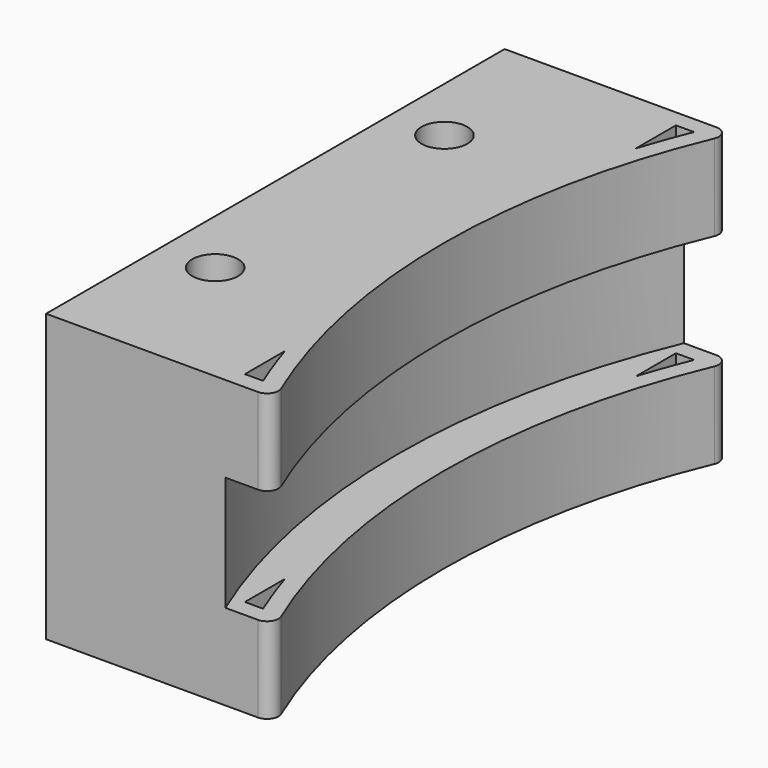
from build123d import *

# Parameters (mm, degrees)
F0_W     = 14.641710973
F0_H     = 25
F0_R     = 2
F2_DEPTH = 25
F1_W     = 8
F1_H     = 10
F4_R     = 1


# Not quite as in the source:
# - a feature names something its author has since deleted; it is built from what else it names


with BuildPart() as f2:
    # F0 (on Top) → F2 (new body)
    with BuildSketch(Plane.XY):
        with BuildLine():
            ThreePointArc((-61, 0), (-59.6453869522, 12.7838888967), (-55.641710973, 25))
            Line((-55.641710973, 25), (-61, 25))
            Line((-61, 25), (-61, 0))
        make_face()
        with BuildLine():
            Line((-59.5, 19.1311264697), (-59.5, 23.5))
            Line((-59.5, 23.5), (-57.9137289423, 23.5))
            ThreePointArc((-57.9137289423, 23.5), (-58.7474910104, 21.3303141089), (-59.5, 19.1311264697))
        make_face(mode=Mode.SUBTRACT)
        with BuildLine():
            ThreePointArc((-55.641710973, -25), (-59.6453869522, -12.7838888967), (-61, 0))
            Line((-61, 0), (-61, -25))
            Line((-61, -25), (-55.641710973, -25))
        make_face()
        with BuildLine():
            Line((-57.9137289423, -23.5), (-59.5, -23.5))
            Line((-59.5, -23.5), (-59.5, -19.1311264697))
            ThreePointArc((-59.5, -19.1311264697), (-58.7474910104, -21.3303141089), (-57.9137289423, -23.5))
        make_face(mode=Mode.SUBTRACT)
        with Locations((-68.3208554865, -12.5)):
            Rectangle(F0_W, F0_H)
        with Locations((-70.891710973, -12.5)):
            Circle(F0_R, mode=Mode.SUBTRACT)
        with Locations((-68.3208554865, 12.5)):
            Rectangle(F0_W, F0_H)
        with Locations((-70.891710973, 12.5)):
            Circle(F0_R, mode=Mode.SUBTRACT)
    extrude(amount=F2_DEPTH)

    # F1 (on Front) → F3 (revolve, cut)
    with BuildSketch(Plane.XZ):
        with Locations((-61, 12.5)):
            Rectangle(F1_W, F1_H)
    revolve(axis=Axis((0, 0, 15.2043728158), (0, 0, 1)), mode=Mode.SUBTRACT)

    # F4
    f4_edges = [f2.edges().sort_by_distance(p)[0] for p in [
        (-55.641711, 25, 21.25),
        (-55.641711, 25, 3.75),
        (-55.641711, -25, 3.75),
        (-55.641711, -25, 21.25),
    ]]
    fillet(f4_edges, radius=F4_R)


solid = f2.part
